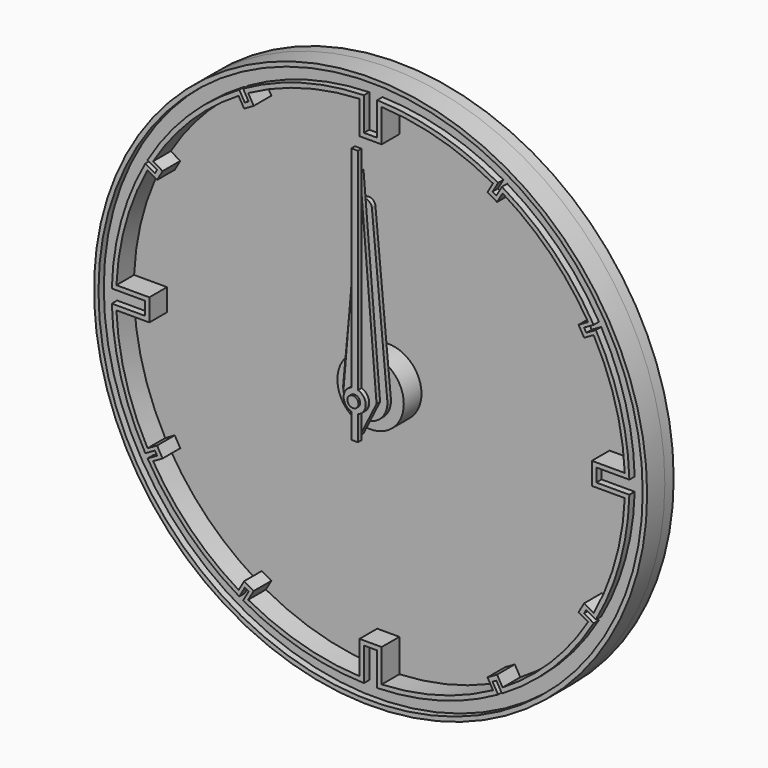
from build123d import *

# Parameters (mm, degrees)
F0_R      = 125
F1_DEPTH  = 5
F2_R      = 15
F3_DEPTH  = 10
F4_R      = 2.5
F5_DEPTH  = 10
F6_R      = 125
F6_R_2    = 115
F7_DEPTH  = 10
F8_W      = 10
F8_H      = 20
F8_W_2    = 20
F8_H_2    = 10
F9_DEPTH  = 10
F11_DEPTH = 10
F12_R     = 123
F12_R_2   = 117
F13_DEPTH = 3
F14_W     = 6
F14_H     = 18
F14_W_2   = 18
F14_H_2   = 6
F15_DEPTH = 3
F17_DEPTH = 3
F19_R     = 2.5
F20_DEPTH = 2
F22_R     = 2.5
F23_DEPTH = 2
F25_R     = 2.5
F26_DEPTH = 2


with BuildPart() as f1:
    # F0 (on Front) → F1 (new body)
    with BuildSketch(Plane.XZ):
        Circle(F0_R)
    extrude(amount=-F1_DEPTH)


with BuildPart() as f3:
    # F2 (on face) → F3 (new body)
    with BuildSketch(Plane.XZ):
        Circle(F2_R)
    extrude(amount=F3_DEPTH)

    # F4 (on face) → F5 (join)
    with BuildSketch(Plane.XZ.offset(10)):
        Circle(F4_R)
    extrude(amount=F5_DEPTH)


with BuildPart() as f7:
    # F6 (on face) → F7 (new body)
    with BuildSketch(Plane.XZ):
        Circle(F6_R)
        Circle(F6_R_2, mode=Mode.SUBTRACT)
    extrude(amount=F7_DEPTH)

    # F8 (on face) → F9 (join)
    with BuildSketch(Plane.XZ):
        with Locations((0, 110)):
            Rectangle(F8_W, F8_H)
        with Locations((-110, 0)):
            Rectangle(F8_W_2, F8_H_2)
        with Locations((0, -110)):
            Rectangle(F8_W, F8_H)
        with Locations((110, 0)):
            Rectangle(F8_W_2, F8_H_2)
    extrude(amount=F9_DEPTH)

    # F10 (on face) → F11 (join)
    with BuildSketch(Plane.XZ):
        Polygon((62.1650635095, 102.6730484541), (57.8349364905, 105.1730484541), (52.8349364905, 96.5127944163), (57.1650635095, 94.0127944163), align=None)
        Polygon((105.1730484541, 57.8349364905), (102.6730484541, 62.1650635095), (94.0127944163, 57.1650635095), (96.5127944163, 52.8349364905), align=None)
        Polygon((-102.6730484541, 62.1650635095), (-105.1730484541, 57.8349364905), (-96.5127944163, 52.8349364905), (-94.0127944163, 57.1650635095), align=None)
        Polygon((-57.8349364905, 105.1730484541), (-62.1650635095, 102.6730484541), (-57.1650635095, 94.0127944163), (-52.8349364905, 96.5127944163), align=None)
        Polygon((-62.1650635095, -102.6730484541), (-57.8349364905, -105.1730484541), (-52.8349364905, -96.5127944163), (-57.1650635095, -94.0127944163), align=None)
        Polygon((-105.1730484541, -57.8349364905), (-102.6730484541, -62.1650635095), (-94.0127944163, -57.1650635095), (-96.5127944163, -52.8349364905), align=None)
        Polygon((102.6730484541, -62.1650635095), (105.1730484541, -57.8349364905), (96.5127944163, -52.8349364905), (94.0127944163, -57.1650635095), align=None)
        Polygon((57.8349364905, -105.1730484541), (62.1650635095, -102.6730484541), (57.1650635095, -94.0127944163), (52.8349364905, -96.5127944163), align=None)
    extrude(amount=F11_DEPTH)

    # F12 (on face) → F13 (cut)
    with BuildSketch(Plane.XZ.offset(10)):
        Circle(F12_R)
        Circle(F12_R_2, mode=Mode.SUBTRACT)
    extrude(amount=-F13_DEPTH, mode=Mode.SUBTRACT)

    # F14 (on face) → F15 (cut)
    with BuildSketch(Plane.XZ.offset(10)):
        with Locations((0, 111)):
            Rectangle(F14_W, F14_H)
        with Locations((-111, 0)):
            Rectangle(F14_W_2, F14_H_2)
        with Locations((0, -111)):
            Rectangle(F14_W, F14_H)
        with Locations((111, 0)):
            Rectangle(F14_W_2, F14_H_2)
    extrude(amount=-F15_DEPTH, mode=Mode.SUBTRACT)

    # F16 (on face) → F17 (cut)
    with BuildSketch(Plane.XZ.offset(10)):
        Polygon((60.142679841, 102.1701771879), (58.4106290334, 103.1701771879), (55.1339745962, 97.4948452239), (56.8660254038, 96.4948452239), align=None)
        Polygon((103.1701771879, 58.4106290334), (102.1701771879, 60.142679841), (96.4948452239, 56.8660254038), (97.4948452239, 55.1339745962), align=None)
        Polygon((-55.1339745962, 97.4948452239), (-58.4106290334, 103.1701771879), (-60.142679841, 102.1701771879), (-56.8660254038, 96.4948452239), align=None)
        Polygon((-96.4948452239, 56.8660254038), (-102.1701771879, 60.142679841), (-103.1701771879, 58.4106290334), (-97.4948452239, 55.1339745962), align=None)
        Polygon((-97.4948452239, -55.1339745962), (-103.1701771879, -58.4106290334), (-102.1701771879, -60.142679841), (-96.4948452239, -56.8660254038), align=None)
        Polygon((-56.8660254038, -96.4948452239), (-60.142679841, -102.1701771879), (-58.4106290334, -103.1701771879), (-55.1339745962, -97.4948452239), align=None)
        Polygon((55.1339745962, -97.4948452239), (58.4106290334, -103.1701771879), (60.142679841, -102.1701771879), (56.8660254038, -96.4948452239), align=None)
        Polygon((96.4948452239, -56.8660254038), (102.1701771879, -60.142679841), (103.1701771879, -58.4106290334), (97.4948452239, -55.1339745962), align=None)
    extrude(amount=-F17_DEPTH, mode=Mode.SUBTRACT)


with BuildPart() as f20:
    # F19 (on offset) → F20 (new body)
    with BuildSketch(Plane.XZ.offset(11)):
        with BuildLine():
            ThreePointArc((2.9869047524, 75.28), (0, 78), (-2.9869047524, 75.28))
            Line((-2.9869047524, 75.28), (-9.9563491747, 0.9333333333))
            ThreePointArc((-9.9563491747, 0.9333333333), (0, -10), (9.9563491747, 0.9333333333))
            Line((9.9563491747, 0.9333333333), (2.9869047524, 75.28))
        make_face()
        Circle(F19_R, mode=Mode.SUBTRACT)
    extrude(amount=F20_DEPTH)


with BuildPart() as f23:
    # F22 (on offset) → F23 (new body)
    with BuildSketch(Plane.XZ.offset(14)):
        Polygon((7.5, 0), (0, 90), (-7.5, 0), (0, -15), align=None)
        Circle(F22_R, mode=Mode.SUBTRACT)
    extrude(amount=F23_DEPTH)


with BuildPart() as f26:
    # F25 (on offset) → F26 (new body)
    with BuildSketch(Plane.XZ.offset(17)):
        with BuildLine():
            Line((1.5, -16), (1.5, -4.7696960071))
            ThreePointArc((1.5, -4.7696960071), (5, 0), (1.5, 4.7696960071))
            Line((1.5, 4.7696960071), (1.5, 100))
            Line((1.5, 100), (-1.5, 100))
            Line((-1.5, 100), (-1.5, 4.7696960071))
            ThreePointArc((-1.5, 4.7696960071), (-5, 0), (-1.5, -4.7696960071))
            Line((-1.5, -4.7696960071), (-1.5, -16))
            Line((-1.5, -16), (1.5, -16))
        make_face()
        Circle(F25_R, mode=Mode.SUBTRACT)
    extrude(amount=F26_DEPTH)


solid = Compound([f1.part, f3.part, f7.part, f20.part, f23.part, f26.part])
